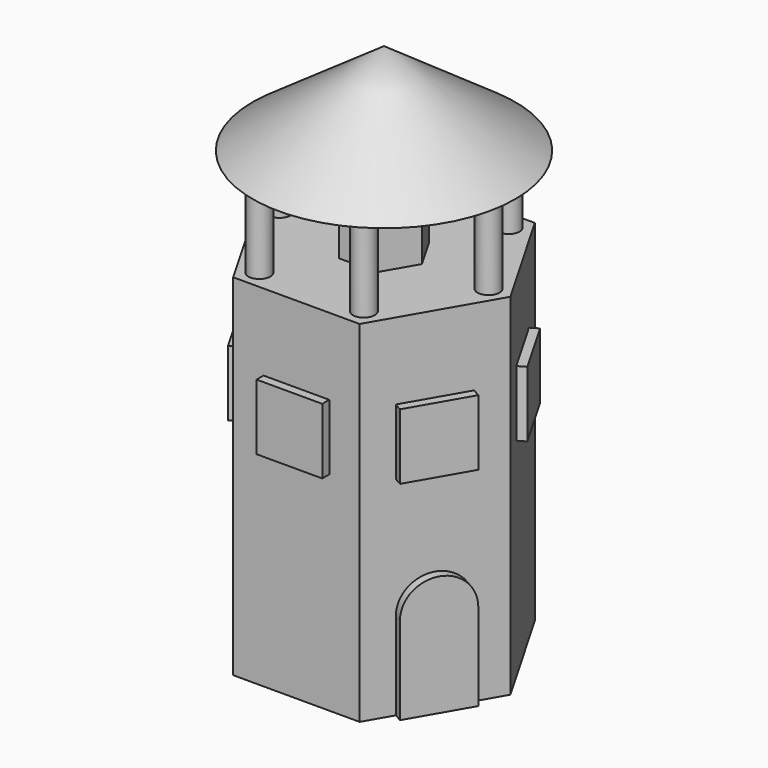
from build123d import *

# Parameters (mm, degrees)
F1_DEPTH        = 80
F2_W            = 15
F2_H            = 15
F3_DEPTH        = 2
F5_COUNT        = 6
F7_DEPTH        = 20
F8_R            = 2.5
F9_DEPTH        = 20
F9_COPIES_COUNT = 6
F12_DEPTH       = 2
F13_R           = 30
F14_DEPTH       = 25
F14_TAPER       = 55


# Not quite as in the source:
# - a pattern or mirror of a feature is missing from the dataset's text; its kind, count and spacing are read off the source's solid


with BuildPart() as f1:
    # F0 (on Top) → F1 (new body)
    with BuildSketch(Plane.XY):
        Polygon((-14.4337567297, -25), (14.4337567297, -25), (28.8675134595, 0), (14.4337567297, 25), (-14.4337567297, 25), (-28.8675134595, 0), align=None)
    extrude(amount=F1_DEPTH)

    # F8 (on face) → F9 (join)
    with BuildSketch(Plane.XY.offset(80)):
        with Locations((-23.8675134595, 0)):
            Circle(F8_R)
    f9 = extrude(amount=F9_DEPTH)

    # F9_copies: F9 ×6 about axis
    f9_copies_axis = Axis((0, 0, 0), (0, 0, 1))
    for i in range(1, F9_COPIES_COUNT):
        add(f9.rotate(f9_copies_axis, i * 360 / F9_COPIES_COUNT))


with BuildPart() as f3:
    # F2 (on face) → F3 (new body)
    with BuildSketch(Plane.XZ.offset(25)):
        with Locations((0, 55)):
            Rectangle(F2_W, F2_H)
    extrude(amount=F3_DEPTH)


with BuildPart() as f5_1:
    # F5: instance of F3
    add(f3.part.rotate(Axis((0, 0, 80), (0, 0, 1)), 1 * 360 / F5_COUNT))


with BuildPart() as f5_2:
    # F5: instance of F3
    add(f3.part.rotate(Axis((0, 0, 80), (0, 0, 1)), 2 * 360 / F5_COUNT))


with BuildPart() as f5_3:
    # F5: instance of F3
    add(f3.part.rotate(Axis((0, 0, 80), (0, 0, 1)), 3 * 360 / F5_COUNT))


with BuildPart() as f5_4:
    # F5: instance of F3
    add(f3.part.rotate(Axis((0, 0, 80), (0, 0, 1)), 4 * 360 / F5_COUNT))


with BuildPart() as f5_5:
    # F5: instance of F3
    add(f3.part.rotate(Axis((0, 0, 80), (0, 0, 1)), 5 * 360 / F5_COUNT))


with BuildPart() as f7:
    # F6 (on face) → F7 (new body)
    with BuildSketch(Plane.XY.offset(80)):
        Polygon((-4.3301270189, -7.5), (4.3301270189, -7.5), (8.6602540378, 0), (4.3301270189, 7.5), (-4.3301270189, 7.5), (-8.6602540378, 0), align=None)
    extrude(amount=F7_DEPTH)


with BuildPart() as f12:
    # F11 (on face) → F12 (new body)
    with BuildSketch(Plane(origin=(21.6506350946, -12.5, 0), x_dir=(0.5, 0.8660254038, 0), z_dir=(0.8660254038, -0.5, 0))):
        with BuildLine():
            Line((7.5, 0), (7.5, 20))
            ThreePointArc((7.5, 20), (0, 27.5), (-7.5, 20))
            Line((-7.5, 20), (-7.5, 0))
            Line((-7.5, 0), (7.5, 0))
        make_face()
    extrude(amount=F12_DEPTH)


with BuildPart() as f14:
    # F13 (on face) → F14 (new body)
    with BuildSketch(Plane.XY.offset(100)):
        Circle(F13_R)
    extrude(amount=F14_DEPTH, taper=F14_TAPER)


solid = Compound([f1.part, f3.part, f5_1.part, f5_2.part, f5_3.part, f5_4.part, f5_5.part, f7.part, f12.part, f14.part])
